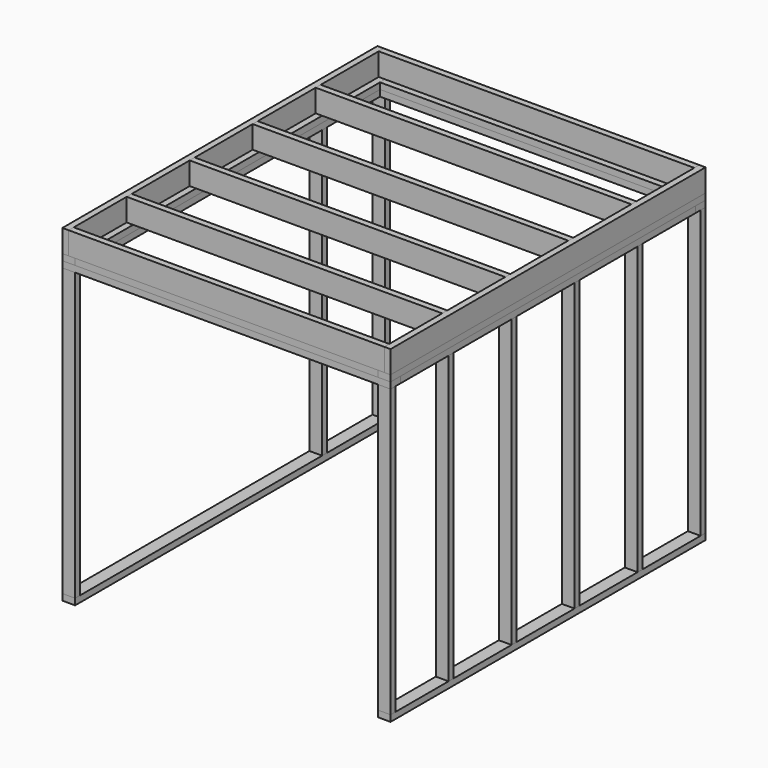
from build123d import *

# Parameters (mm, degrees)
F3_W      = 48
F3_H      = 3000
F4_DEPTH  = 172
F5_W      = 2404
F5_H      = 48
F6_DEPTH  = 172
F7_W      = 97
F7_H      = 3000
F8_DEPTH  = 48
F9_W      = 2306
F9_H      = 97
F10_DEPTH = 48
F11_W     = 2500
F11_H     = 97
F12_DEPTH = 48
F13_W     = 97
F13_H     = 2806
F14_DEPTH = 48
F15_W     = 3000
F15_H     = 48
F16_DEPTH = 97
F17_W     = 48
F17_H     = 2184
F18_DEPTH = 97
F19_W     = 3000
F19_H     = 48
F20_DEPTH = 97
F21_W     = 48
F21_H     = 2184
F22_DEPTH = 97
F23_W     = 48
F23_H     = 2184
F24_DEPTH = 97


with BuildPart() as f4:
    # F3 (on Top) → F4 (new body)
    with BuildSketch(Plane.XY):
        with Locations((-24, -1500)):
            Rectangle(F3_W, F3_H)
    extrude(amount=-F4_DEPTH)


with BuildPart() as f4b:
    # F3 (on Top) → F4, piece 2 (new body)
    with BuildSketch(Plane.XY):
        with Locations((-2476, -1500)):
            Rectangle(F3_W, F3_H)
    extrude(amount=-F4_DEPTH)


with BuildPart() as f6:
    # F5 (on face) → F6 (new body)
    with BuildSketch(Plane.XY):
        with Locations((-1250, -24)):
            Rectangle(F5_W, F5_H)
    extrude(amount=-F6_DEPTH)


with BuildPart() as f6b:
    # F5 (on face) → F6, piece 2 (new body)
    with BuildSketch(Plane.XY):
        with Locations((-1250, -624)):
            Rectangle(F5_W, F5_H)
    extrude(amount=-F6_DEPTH)


with BuildPart() as f6c:
    # F5 (on face) → F6, piece 3 (new body)
    with BuildSketch(Plane.XY):
        with Locations((-1250, -1224)):
            Rectangle(F5_W, F5_H)
    extrude(amount=-F6_DEPTH)


with BuildPart() as f6d:
    # F5 (on face) → F6, piece 4 (new body)
    with BuildSketch(Plane.XY):
        with Locations((-1250, -1824)):
            Rectangle(F5_W, F5_H)
    extrude(amount=-F6_DEPTH)


with BuildPart() as f6e:
    # F5 (on face) → F6, piece 5 (new body)
    with BuildSketch(Plane.XY):
        with Locations((-1250, -2424)):
            Rectangle(F5_W, F5_H)
    extrude(amount=-F6_DEPTH)


with BuildPart() as f6f:
    # F5 (on face) → F6, piece 6 (new body)
    with BuildSketch(Plane.XY):
        with Locations((-1250, -2976)):
            Rectangle(F5_W, F5_H)
    extrude(amount=-F6_DEPTH)


with BuildPart() as f8:
    # F7 (on face) → F8 (new body)
    with BuildSketch(Plane(origin=(0, 0, -172), x_dir=(1, 0, 0), z_dir=(0, 0, -1))):
        with Locations((-48.5, 1500)):
            Rectangle(F7_W, F7_H)
    extrude(amount=F8_DEPTH)


with BuildPart() as f8b:
    # F7 (on face) → F8, piece 2 (new body)
    with BuildSketch(Plane(origin=(0, 0, -172), x_dir=(1, 0, 0), z_dir=(0, 0, -1))):
        with Locations((-2451.5, 1500)):
            Rectangle(F7_W, F7_H)
    extrude(amount=F8_DEPTH)


with BuildPart() as f10:
    # F9 (on face) → F10 (new body)
    with BuildSketch(Plane(origin=(0, 0, -172), x_dir=(1, 0, 0), z_dir=(0, 0, -1))):
        with Locations((-1250, 48.5)):
            Rectangle(F9_W, F9_H)
    extrude(amount=F10_DEPTH)


with BuildPart() as f10b:
    # F9 (on face) → F10, piece 2 (new body)
    with BuildSketch(Plane(origin=(0, 0, -172), x_dir=(1, 0, 0), z_dir=(0, 0, -1))):
        with Locations((-1250, 2951.5)):
            Rectangle(F9_W, F9_H)
    extrude(amount=F10_DEPTH)


with BuildPart() as f12:
    # F11 (on face) → F12 (new body)
    with BuildSketch(Plane(origin=(0, 0, -220), x_dir=(1, 0, 0), z_dir=(0, 0, -1))):
        with Locations((-1250, 48.5)):
            Rectangle(F11_W, F11_H)
    extrude(amount=F12_DEPTH)


with BuildPart() as f12b:
    # F11 (on face) → F12, piece 2 (new body)
    with BuildSketch(Plane(origin=(0, 0, -220), x_dir=(1, 0, 0), z_dir=(0, 0, -1))):
        with Locations((-1250, 2951.5)):
            Rectangle(F11_W, F11_H)
    extrude(amount=F12_DEPTH)


with BuildPart() as f14:
    # F13 (on face) → F14 (new body)
    with BuildSketch(Plane(origin=(0, 0, -220), x_dir=(1, 0, 0), z_dir=(0, 0, -1))):
        with Locations((-48.5, 1500)):
            Rectangle(F13_W, F13_H)
    extrude(amount=F14_DEPTH)


with BuildPart() as f14b:
    # F13 (on face) → F14, piece 2 (new body)
    with BuildSketch(Plane(origin=(0, 0, -220), x_dir=(1, 0, 0), z_dir=(0, 0, -1))):
        with Locations((-2451.5, 1500)):
            Rectangle(F13_W, F13_H)
    extrude(amount=F14_DEPTH)


with BuildPart() as f16:
    # F15 (on Right) → F16 (new body)
    with BuildSketch(Plane.YZ):
        with Locations((-1500, -2476)):
            Rectangle(F15_W, F15_H)
    extrude(amount=-F16_DEPTH)


with BuildPart() as f18:
    # F17 (on Right) → F18 (new body)
    with BuildSketch(Plane.YZ):
        with Locations((-24, -1360)):
            Rectangle(F17_W, F17_H)
    extrude(amount=-F18_DEPTH)


with BuildPart() as f18b:
    # F17 (on Right) → F18, piece 2 (new body)
    with BuildSketch(Plane.YZ):
        with Locations((-624, -1360)):
            Rectangle(F17_W, F17_H)
    extrude(amount=-F18_DEPTH)


with BuildPart() as f18c:
    # F17 (on Right) → F18, piece 3 (new body)
    with BuildSketch(Plane.YZ):
        with Locations((-1224, -1360)):
            Rectangle(F17_W, F17_H)
    extrude(amount=-F18_DEPTH)


with BuildPart() as f18d:
    # F17 (on Right) → F18, piece 4 (new body)
    with BuildSketch(Plane.YZ):
        with Locations((-1824, -1360)):
            Rectangle(F17_W, F17_H)
    extrude(amount=-F18_DEPTH)


with BuildPart() as f18e:
    # F17 (on Right) → F18, piece 5 (new body)
    with BuildSketch(Plane.YZ):
        with Locations((-2424, -1360)):
            Rectangle(F17_W, F17_H)
    extrude(amount=-F18_DEPTH)


with BuildPart() as f18f:
    # F17 (on Right) → F18, piece 6 (new body)
    with BuildSketch(Plane.YZ):
        with Locations((-2976, -1360)):
            Rectangle(F17_W, F17_H)
    extrude(amount=-F18_DEPTH)


with BuildPart() as f20:
    # F19 (on face) → F20 (new body)
    with BuildSketch(Plane(origin=(-2500, 0, 0), x_dir=(0, -1, 0), z_dir=(-1, 0, 0))):
        with Locations((1500, -2476)):
            Rectangle(F19_W, F19_H)
    extrude(amount=-F20_DEPTH)


with BuildPart() as f22:
    # F21 (on face) → F22 (new body)
    with BuildSketch(Plane(origin=(-2500, 0, 0), x_dir=(0, -1, 0), z_dir=(-1, 0, 0))):
        with Locations((24, -1360)):
            Rectangle(F21_W, F21_H)
    extrude(amount=-F22_DEPTH)


with BuildPart() as f22b:
    # F21 (on face) → F22, piece 2 (new body)
    with BuildSketch(Plane(origin=(-2500, 0, 0), x_dir=(0, -1, 0), z_dir=(-1, 0, 0))):
        with Locations((624, -1360)):
            Rectangle(F21_W, F21_H)
    extrude(amount=-F22_DEPTH)


with BuildPart() as f24:
    # F23 (on face) → F24 (new body)
    with BuildSketch(Plane(origin=(-2500, 0, 0), x_dir=(0, -1, 0), z_dir=(-1, 0, 0))):
        with Locations((2976, -1360)):
            Rectangle(F23_W, F23_H)
    extrude(amount=-F24_DEPTH)


solid = Compound([f4.part, f4b.part, f6.part, f6b.part, f6c.part, f6d.part, f6e.part, f6f.part, f8.part, f8b.part, f10.part, f10b.part, f12.part, f12b.part, f14.part, f14b.part, f16.part, f18.part, f18b.part, f18c.part, f18d.part, f18e.part, f18f.part, f20.part, f22.part, f22b.part, f24.part])
